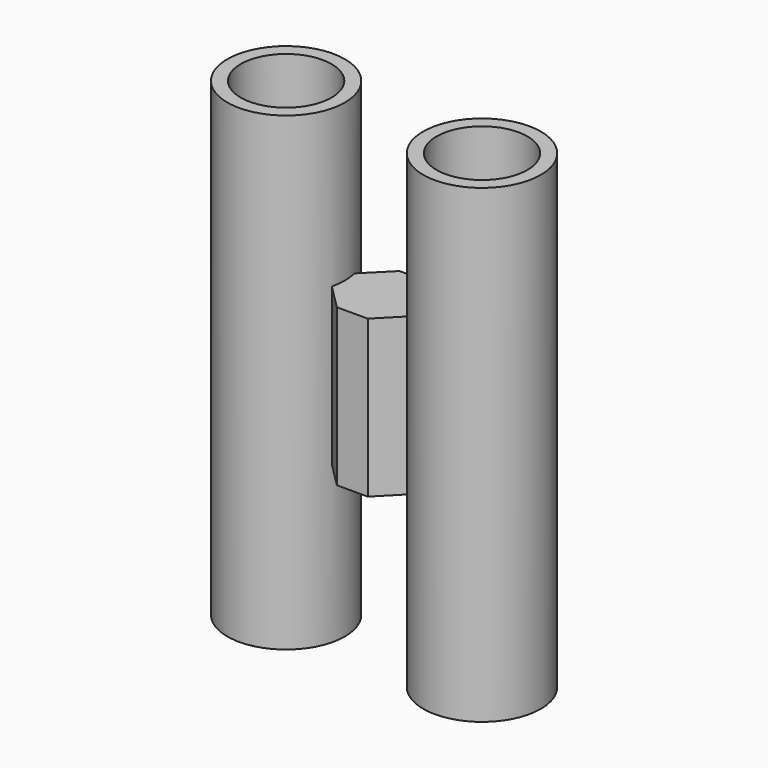
from build123d import *

# Parameters (mm, degrees)
F0_R           = 9.525
F1_DEPTH       = 38.1
F4_W           = 7.6494621422
F4_H           = 6.35
F5_DEPTH       = 12.7
F8_D           = 14.732
F8_DEPTH       = 69.85
F8_TIP         = 4.4259393198
F8_ON_F7_D     = 14.732
F8_ON_F7_DEPTH = 69.85
F8_ON_F7_TIP   = 4.4259393198
F9_T4_DEPTH    = 51.5282991577
F9_S5_R        = 9.525
F9_T6_DEPTH    = 28
F9_T10_DEPTH   = 51.965031671
F9_S11_R       = 9.525
F9_T12_DEPTH   = 28
F9_T16_DEPTH   = 51.965031671
F9_S17_R       = 9.525
F9_T18_DEPTH   = 28
F9_T22_DEPTH   = 51.5282991577
F9_S23_R       = 9.525
F9_T24_DEPTH   = 28


# Not quite as in the source:
# - a fillet or chamfer that OpenCascade refuses, or shapes differently, is made with other operations: its cross-section is extruded or revolved along the edge and cut away or added
# - a feature of the source that left no trace in its solid (it failed there, or was rolled back) is left out


with BuildPart() as f1:
    # F0 (on Top) → F1 (new body, symmetric)
    with BuildSketch(Plane.XY):
        with Locations((-15.875, 0)):
            Circle(F0_R)
    extrude(amount=F1_DEPTH, both=True)



with BuildPart() as f1b:
    # F0 (on Top) → F1, piece 2 (new body, symmetric)
    with BuildSketch(Plane.XY):
        with Locations((15.875, 0)):
            Circle(F0_R)
    extrude(amount=F1_DEPTH, both=True)


with BuildPart() as f1_1:
    add(f1.part)

    add(f1b.part)  # F5 merges F1b
    # F4 (on Top) → F5 (join, symmetric)
    with BuildSketch(Plane.XY):
        with Locations((-3.8247310711, 3.175)):
            Rectangle(F4_W, F4_H)
        Polygon((7.4973143637, 0), (0, 0), (0, -6.35), (7.6071062533, -6.35), align=None)
        Polygon((0, 6.35), (0, 0), (7.4973143637, 0), (7.6071062533, 6.35), align=None)
        with Locations((-3.8247310711, -3.175)):
            Rectangle(F4_W, F4_H)
    extrude(amount=F5_DEPTH, both=True)

    # F8
    with Locations(Plane.XY.offset(38.1)):
        with Locations((-15.875, 0)):
            Hole(F8_D / 2, depth=F8_DEPTH)
            with Locations((0, 0, -(F8_DEPTH + F8_TIP / 2))):  # 118° drill point
                Cone(0, F8_D / 2, F8_TIP, mode=Mode.SUBTRACT)

    # F8 on F7
    with Locations(Plane.XY.offset(38.1)):
        with Locations((15.875, 0)):
            Hole(F8_ON_F7_D / 2, depth=F8_ON_F7_DEPTH)
            with Locations((0, 0, -(F8_ON_F7_DEPTH + F8_ON_F7_TIP / 2))):  # 118° drill point
                Cone(0, F8_ON_F7_D / 2, F8_ON_F7_TIP, mode=Mode.SUBTRACT)

    # F9: chamfer of 5.08 on 4 edges, made by hand


with BuildPart() as f9_tool2:
    # F9_s3 → F9_t4 (new body)
    with BuildSketch(Plane.XY.offset(25.7641495789)):
        Polygon((-7.6494621422, -1.27), (-2.5694621422, -6.35), (-7.6494621422, -6.35), align=None)
    extrude(amount=-F9_T4_DEPTH)

    # F9_s5 → F9_t6 (cut, symmetric)
    with BuildSketch(Plane.XY):
        with Locations((-15.875, 0)):
            Circle(F9_S5_R)
    extrude(amount=F9_T6_DEPTH, both=True, mode=Mode.SUBTRACT)


with BuildPart() as f1_2:
    add(f1_1.part)

    # F9_t1: cut F9_tool2
    add(f9_tool2.part, mode=Mode.SUBTRACT)


with BuildPart() as f9_tool8:
    # F9_s9 → F9_t10 (new body)
    with BuildSketch(Plane.XY.offset(25.9825158355)):
        Polygon((7.5177543218, -1.1821796141), (2.438513475, -6.35), (7.6071062533, -6.35), align=None)
    extrude(amount=-F9_T10_DEPTH)

    # F9_s11 → F9_t12 (cut, symmetric)
    with BuildSketch(Plane.XY):
        with Locations((15.875, 0)):
            Circle(F9_S11_R)
    extrude(amount=F9_T12_DEPTH, both=True, mode=Mode.SUBTRACT)


with BuildPart() as f1_3:
    add(f1_2.part)

    # F9_t7: cut F9_tool8
    add(f9_tool8.part, mode=Mode.SUBTRACT)


with BuildPart() as f9_tool14:
    # F9_s15 → F9_t16 (new body)
    with BuildSketch(Plane.XY.offset(-25.9825158355)):
        Polygon((7.5177543218, 1.1821796141), (2.438513475, 6.35), (7.6071062533, 6.35), align=None)
    extrude(amount=F9_T16_DEPTH)

    # F9_s17 → F9_t18 (cut, symmetric)
    with BuildSketch(Plane.XY):
        with Locations((15.875, 0)):
            Circle(F9_S17_R)
    extrude(amount=F9_T18_DEPTH, both=True, mode=Mode.SUBTRACT)


with BuildPart() as f1_4:
    add(f1_3.part)

    # F9_t13: cut F9_tool14
    add(f9_tool14.part, mode=Mode.SUBTRACT)


with BuildPart() as f9_tool20:
    # F9_s21 → F9_t22 (new body)
    with BuildSketch(Plane.XY.offset(25.7641495789)):
        Polygon((-7.6494621422, 1.27), (-2.5694621422, 6.35), (-7.6494621422, 6.35), align=None)
    extrude(amount=-F9_T22_DEPTH)

    # F9_s23 → F9_t24 (cut, symmetric)
    with BuildSketch(Plane.XY):
        with Locations((-15.875, 0)):
            Circle(F9_S23_R)
    extrude(amount=F9_T24_DEPTH, both=True, mode=Mode.SUBTRACT)


with BuildPart() as f1_5:
    add(f1_4.part)

    # F9_t19: cut F9_tool20
    add(f9_tool20.part, mode=Mode.SUBTRACT)


solid = f1_5.part
